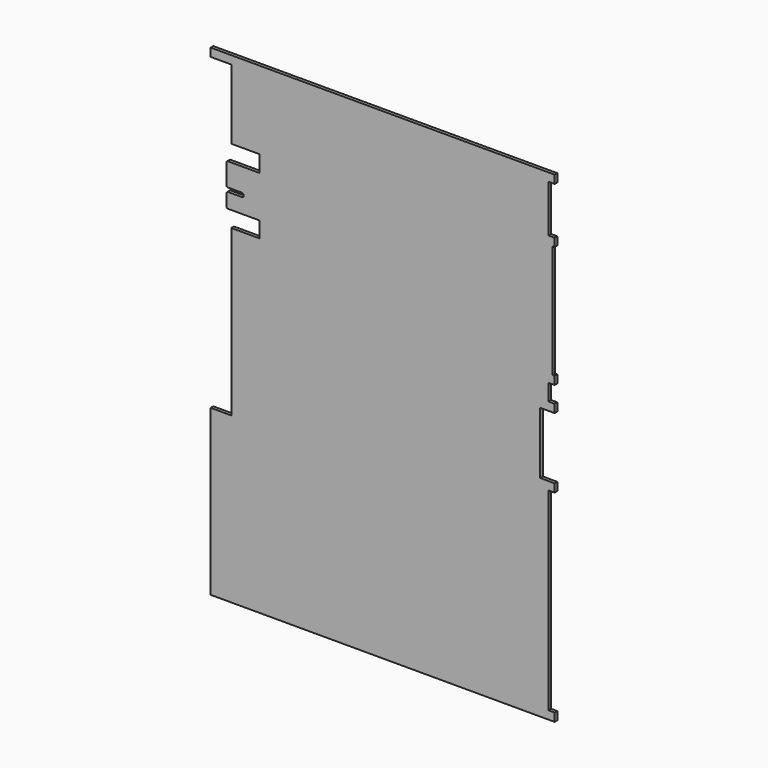
from build123d import *

# Parameters (mm, degrees)
F0_W     = 10.2457383797
F0_H     = 20.3
F0_W_2   = 2.4
F0_H_2   = 7.2
F0_H_3   = 11.2
F1_DEPTH = 1.6
F2_SIZE  = 0.5
F3_R     = 0.94999


# Not quite as in the source:
# - a fillet or chamfer is up to 0.001 mm smaller than in the source, because OpenCascade refuses the exact size


with BuildPart() as f1:
    # F0 (on Front) → F1 (new body)
    with BuildSketch(Plane.XZ):
        Polygon((0, 79.96), (0, 0), (167, 0), (167, 4), (164, 4), (164, 98), (167, 98), (167, 102), (160, 102), (160, 132), (167, 132), (167, 136), (164, 136), (164, 144), (167, 144), (167, 147.96), (166, 147.96), (166, 202.96), (167, 202.96), (167, 206.96), (164, 206.96), (164, 229.96), (167, 229.96), (167, 233.96), (0, 233.96), (0, 229.96), (10, 229.96), (10, 196.0979268551), (23.6, 196.0979268551), (23.6, 188.0729268551), (33.8457383797, 188.0729268551), (33.8457383797, 167.7729268551), (23.6, 167.7729268551), (23.6, 160.0979268551), (10, 160.0979268551), (10, 79.96), align=None)
        with Locations((28.7228691898, 177.9229268551)):
            Rectangle(F0_W, F0_H)
        Polygon((10, 174.9729268551), (10, 167.7729268551), (23.6, 167.7729268551), (23.6, 188.0729268551), (10, 188.0729268551), (10, 176.8729268551), (16, 176.8729268551), (16, 174.9729268551), align=None)
        with Locations((8.8, 171.3729268551)):
            Rectangle(F0_W_2, F0_H_2)
        with Locations((8.8, 182.4729268551)):
            Rectangle(F0_W_2, F0_H_3)
    extrude(amount=F1_DEPTH)

    # F2
    f2_edges = [f1.edges().sort_by_distance(p)[0] for p in [
        (7.6, -0.8, 167.772927),
        (7.6, -0.8, 174.972927),
        (7.6, -0.8, 176.872927),
        (7.6, -0.8, 188.072927),
    ]]
    chamfer(f2_edges, length=F2_SIZE)

    # F3 (radius 0.95 in the source; OpenCascade refuses exactly that, so slightly less here)
    f3_edges = [f1.edges().sort_by_distance(p)[0] for p in [
        (16, -0.8, 176.872927),
        (16, -0.8, 174.972927),
    ]]
    fillet(f3_edges, radius=F3_R)


solid = f1.part
